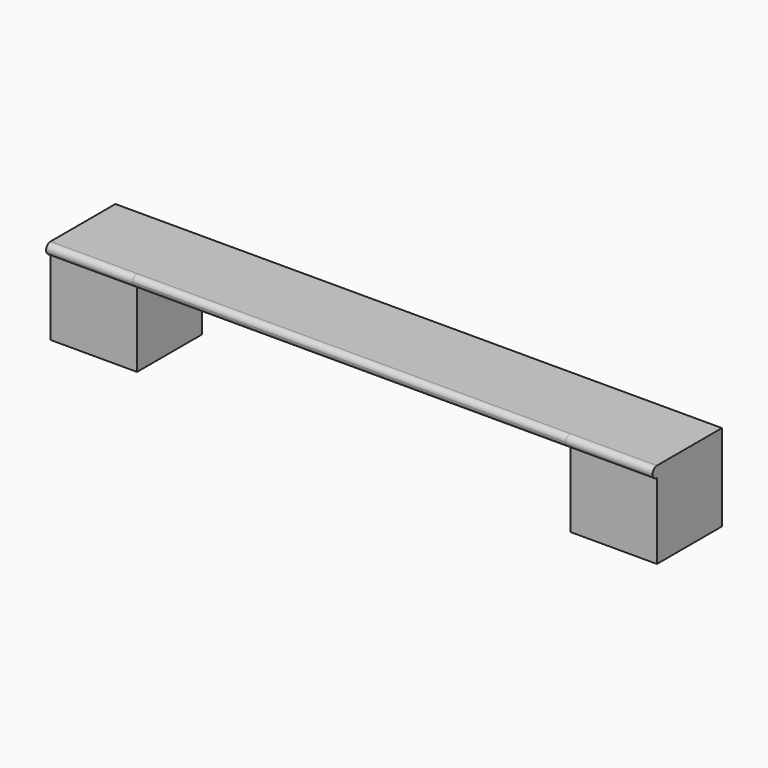
from build123d import *

# Parameters (mm, degrees)
F0_W     = 50.8
F0_H     = 6.35
F1_DEPTH = 254
F2_R     = 3.17499
F3_W     = 47.625
F3_H     = 50.8
F4_DEPTH = 50.8
F6_DEPTH = 50.8
F8_DEPTH = 50.8


# Not quite as in the source:
# - a fillet or chamfer is up to 0.001 mm smaller than in the source, because OpenCascade refuses the exact size


with BuildPart() as f1:
    # F0 (on Right) → F1 (new body)
    with BuildSketch(Plane.YZ):
        Rectangle(F0_W, F0_H)
    extrude(amount=F1_DEPTH)

    # F2 (radius 3.175 in the source; OpenCascade refuses exactly that, so slightly less here)
    f2_edges = [f1.edges().sort_by_distance(p)[0] for p in [
        (127, -25.4, 3.175),
        (127, -25.4, -3.175),
    ]]
    fillet(f2_edges, radius=F2_R)

    # F3 (on face) → F4 (join)
    with BuildSketch(Plane(origin=(0, 0, 0), x_dir=(0, -1, 0), z_dir=(-1, 0, 0))):
        with Locations((-1.5875, -22.225)):
            Rectangle(F3_W, F3_H)
    extrude(amount=F4_DEPTH)

    # F5 (on face) → F6 (join, through all)
    with BuildSketch(Plane(origin=(0, 0, 0), x_dir=(0, -1, 0), z_dir=(-1, 0, 0))):
        with BuildLine():
            Line((22.225, 3.175), (22.225, -3.175))
            ThreePointArc((22.225, -3.175), (25.4, 0), (22.225, 3.175))
        make_face()
    extrude(amount=F6_DEPTH)

    # F7 (on face) → F8 (join)
    with BuildSketch(Plane.YZ.offset(254)):
        with BuildLine():
            Line((-22.225, -3.175), (-22.225, -47.625))
            Line((-22.225, -47.625), (25.4, -47.625))
            Line((25.4, -47.625), (25.4, 3.175))
            Line((25.4, 3.175), (-22.225, 3.175))
            ThreePointArc((-22.225, 3.175), (-25.4, 0), (-22.225, -3.175))
        make_face()
    extrude(amount=F8_DEPTH)


solid = f1.part
